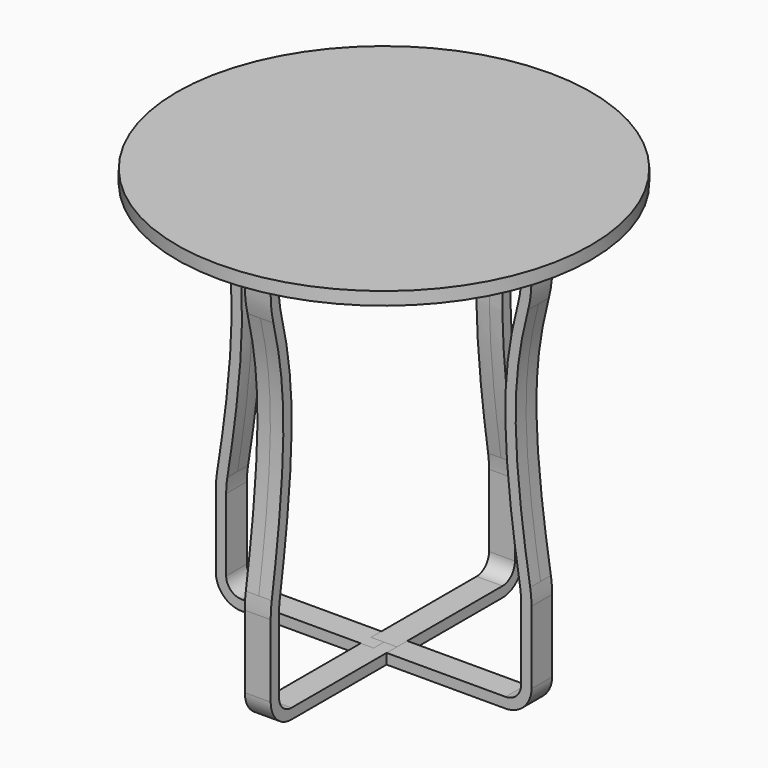
from build123d import *

# Parameters (mm, degrees)
F1_R     = 400
F2_DEPTH = 25
F4_DEPTH = 25
F5_COUNT = 4


# Not quite as in the source:
# - ends of sketch curves that miss each other by under 0.0002 mm in the source are joined
# - the dataset's text gives a spline's control points without its knots; the knots are read off the source's solid


with BuildPart() as f2:
    # F1 (on offset) → F2 (new body)
    with BuildSketch(Plane.XY.offset(800)):
        Circle(F1_R)
    extrude(amount=F2_DEPTH)


with BuildPart() as f4:
    # F3 (on Front) → F4 (new body, symmetric)
    with BuildSketch(Plane.XZ):
        with BuildLine():
            Line((0, 20), (0, 0))
            Line((0, 0), (254.7462901879, 0))
            ThreePointArc((254.7462901879, 0), (290.1016292472, 14.6446609407), (304.7462901879, 50))
            Line((304.7462901879, 50), (304.7462901879, 190.0418571328))
            ThreePointArc((304.7462901879, 190.0418571328), (304.124635747, 205.7986119419), (302.2635369667, 221.4574141851))
            add(Edge.make_bspline(
                [(298.2439789353, 691.7988266907), (286.6172571709, 647.3225839964), (263.1144998863, 519.9412796692), (283.2661495138, 340.8986088594), (302.2635369667, 221.4574141851)],
                knots=[0.1864568588, 0.1864568588, 0.1864568588, 0.1864568588, 0.4082296984, 0.7774710106, 0.7774710106, 0.7774710106, 0.7774710106], degree=3))
            ThreePointArc((298.2439789353, 691.7988266907), (303.1140518699, 716.8822418648), (304.7462901879, 742.3818717691))
            Line((304.7462901879, 742.3818717691), (304.7462901879, 799.2827296257))
            Line((304.7462901879, 799.2827296257), (284.7462901879, 799.2827296257))
            Line((284.7462901879, 799.2827296257), (284.7462901879, 742.3818717691))
            ThreePointArc((284.7462901879, 742.3818717691), (283.2772757017, 719.4322048552), (278.8942100606, 696.8571311986))
            add(Edge.make_bspline(
                [(278.8942100606, 696.8571311986), (278.8382940961, 696.6432366939), (275.4359572991, 683.6086373766), (270.7002052302, 663.6925273568), (265.3629555608, 636.2743171731), (261.8748672485, 615.0745182929), (258.9620620085, 593.180693678), (257.0636577341, 574.3091459077), (255.8916250441, 558.807748383), (255.1928416093, 546.9705765534), (254.6826483373, 534.9223408055), (254.2488970995, 518.6060342435), (254.1532726832, 497.7393771097), (254.709004779, 471.9858426486), (255.892206776, 445.5562931349), (258.2507316117, 409.4684029644), (262.5602812672, 362.8677824804), (269.5883073285, 304.8929298204), (276.5561790639, 256.3560473507), (281.0918124557, 227.2437147341), (282.5118065364, 218.315857565)],
                knots=[0.1864568583, 0.1864568583, 0.1864568583, 0.1864568583, 0.1875, 0.25, 0.28125, 0.3125, 0.34375, 0.375, 0.390625, 0.40625, 0.421875, 0.4375, 0.46875, 0.5, 0.53125, 0.5625, 0.625, 0.6875, 0.75, 0.777470994, 0.777470994, 0.777470994, 0.777470994], degree=3))
            ThreePointArc((282.5118065364, 218.315857565), (284.1868011911, 204.222936461), (284.7462901879, 190.0418571328))
            Line((284.7462901879, 190.0418571328), (284.7462901879, 50))
            ThreePointArc((284.7462901879, 50), (275.9594936235, 28.7867965644), (254.7462901879, 20))
            Line((254.7462901879, 20), (0, 20))
        make_face()
    extrude(amount=F4_DEPTH, both=True)


with BuildPart() as f5_1:
    # F5: instance of F4
    add(f4.part.rotate(Axis((0, 0, 800), (0, 0, -1)), 1 * 360 / F5_COUNT))


with BuildPart() as f5_2:
    # F5: instance of F4
    add(f4.part.rotate(Axis((0, 0, 800), (0, 0, -1)), 2 * 360 / F5_COUNT))


with BuildPart() as f5_3:
    # F5: instance of F4
    add(f4.part.rotate(Axis((0, 0, 800), (0, 0, -1)), 3 * 360 / F5_COUNT))


solid = Compound([f2.part, f4.part, f5_1.part, f5_2.part, f5_3.part])
